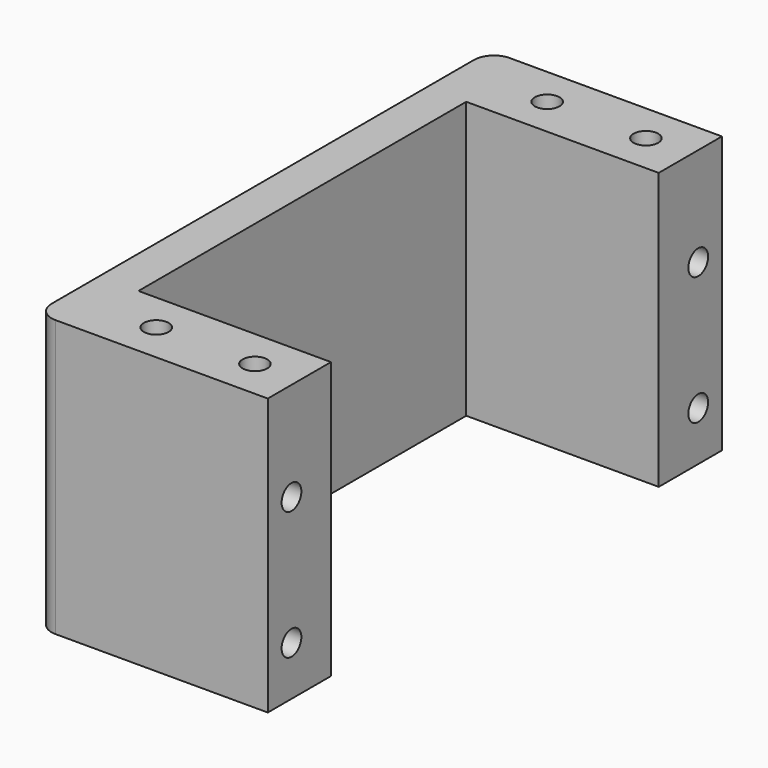
from build123d import *

# Parameters (mm, degrees)
F0_R        = 1.25
F1_DEPTH    = 28
F2_R        = 1.25
F3_DEPTH    = 23.501
F4_T1_DEPTH = 38


# Not quite as in the source:
# - a fillet or chamfer that OpenCascade refuses, or shapes differently, is made with other operations: its cross-section is extruded or revolved along the edge and cut away or added


with BuildPart() as f1:
    # F0 (on Top) → F1 (new body)
    with BuildSketch(Plane.XY):
        Polygon((-19.5, 20.75), (0, 20.75), (0, 28.75), (-23.5, 28.75), (-23.5, -28.75), (0, -28.75), (0, -20.75), (-19.5, -20.75), align=None)
        with Locations((-14.5, -24.75)):
            Circle(F0_R, mode=Mode.SUBTRACT)
        with Locations((-4.5, -24.75)):
            Circle(F0_R, mode=Mode.SUBTRACT)
        with Locations((-14.5, 24.75)):
            Circle(F0_R, mode=Mode.SUBTRACT)
        with Locations((-4.5, 24.75)):
            Circle(F0_R, mode=Mode.SUBTRACT)
    extrude(amount=-F1_DEPTH)

    # F2 (on face) → F3 (cut, through all)
    with BuildSketch(Plane.YZ):
        with Locations((-25.75, -10)):
            Circle(F2_R)
        with Locations((-25.75, -23)):
            Circle(F2_R)
        with Locations((25.75, -10)):
            Circle(F2_R)
        with Locations((25.75, -23)):
            Circle(F2_R)
    extrude(amount=-F3_DEPTH, mode=Mode.SUBTRACT)

    # F4: fillet of radius 2 on 2 edges, made by hand

    # F4_s2 → F4_t1 (cut)
    with BuildSketch(Plane.XY.offset(-33)):
        with BuildLine():
            ThreePointArc((-23.5, -26.75), (-22.9142135624, -28.1642135624), (-21.5, -28.75))
            Line((-21.5, -28.75), (-23.5, -28.75))
            Line((-23.5, -28.75), (-23.5, -26.75))
        make_face()
        with BuildLine():
            ThreePointArc((-21.5, 28.75), (-22.9142135624, 28.1642135624), (-23.5, 26.75))
            Line((-23.5, 26.75), (-23.5, 28.75))
            Line((-23.5, 28.75), (-21.5, 28.75))
        make_face()
    extrude(amount=F4_T1_DEPTH, mode=Mode.SUBTRACT)


solid = f1.part
